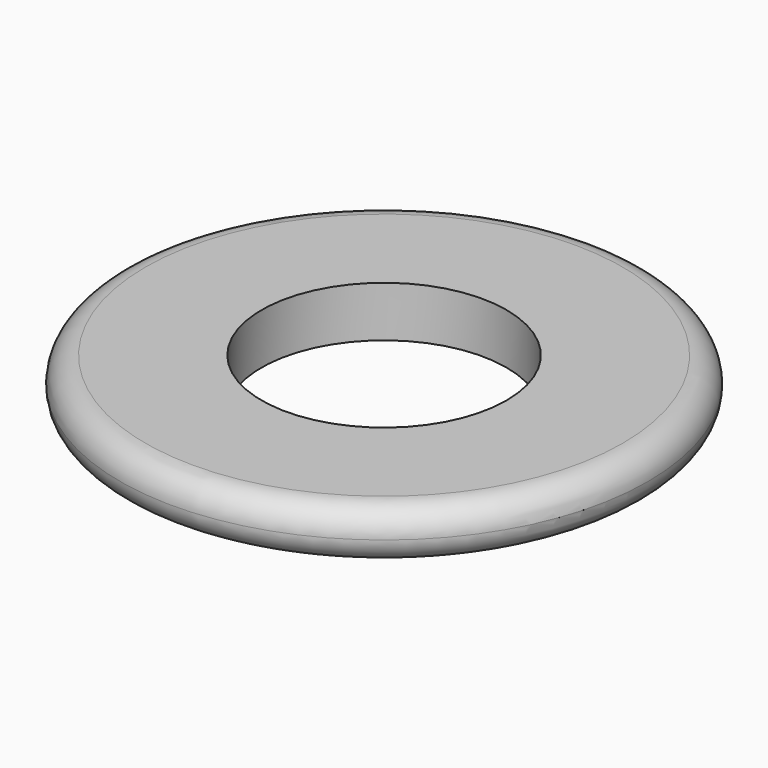
from build123d import *

# Parameters (mm, degrees)
F0_R     = 7.9375
F0_R_2   = 3.683
F1_DEPTH = 1.524
F2_R     = 0.76199


# Not quite as in the source:
# - a fillet or chamfer is up to 0.001 mm smaller than in the source, because OpenCascade refuses the exact size


with BuildPart() as f1:
    # F0 (on Top) → F1 (new body)
    with BuildSketch(Plane.XY):
        Circle(F0_R)
        Circle(F0_R_2, mode=Mode.SUBTRACT)
    extrude(amount=F1_DEPTH)

    # F2 (radius 0.762 in the source; OpenCascade refuses exactly that, so slightly less here)
    f2_edges = [f1.edges().sort_by_distance(p)[0] for p in [
        (-7.9375, 0, 1.524),
        (-7.9375, 0, 0),
    ]]
    fillet(f2_edges, radius=F2_R)


solid = f1.part
